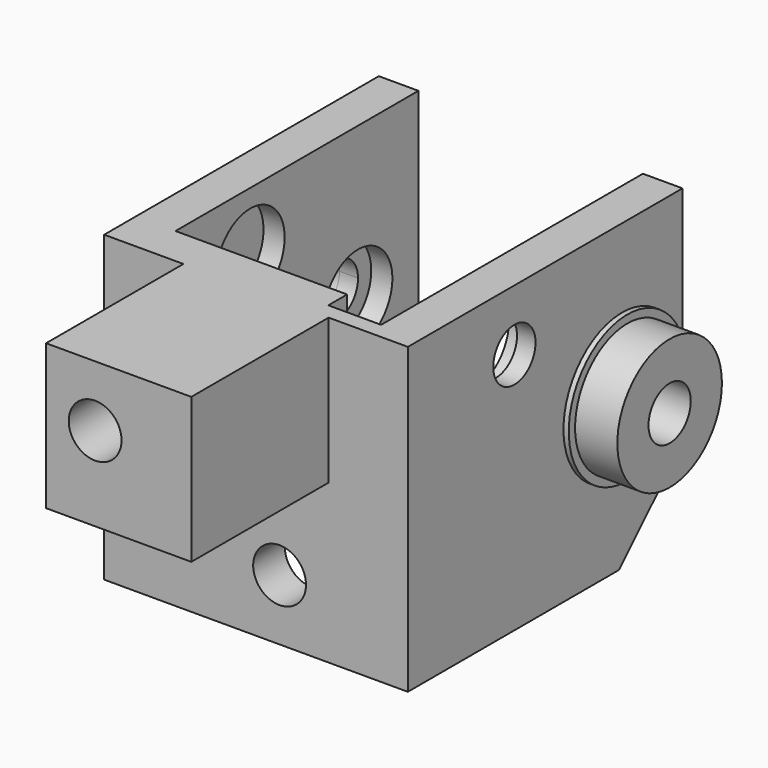
from build123d import *
from build123d import SkipClean  # not in build123d's __all__

# Parameters (mm, degrees)
F1_W             = 115
F1_H             = 115
F2_DEPTH         = 15
F5_W             = 100
F5_H             = 115
F5_R             = 10
F6_DEPTH         = 25
F4_W             = 115
F4_H             = 115
F4_R             = 10
F6_FACE_W        = 25
F6_FACE_H        = 115
F7_DEPTH         = 15
F8_R             = 24.75
F8_R_2           = 10
F9_DEPTH         = 18
F10_SIZE         = 30
F11_R            = 27.75
F11_R_2          = 24.75
F12_DEPTH        = 2
F14_R            = 16.25
F15_DEPTH        = 8
F15_COPIES_COUNT = 2
F15_COPIES_PITCH = 93
F16_R            = 50
F17_DEPTH        = 20
F18_R            = 50
F19_DEPTH        = 20
F20_W            = 115
F20_H            = 115
F20_R            = 10
F21_DEPTH        = 55
F22_W            = 55
F22_H            = 60
F22_R            = 10
F23_DEPTH        = 65


# Not quite as in the source:
# - after a boolean that leaves OpenCascade's solid faulty, fix() repairs it
# - a pattern or mirror of a feature is missing from the dataset's text; its kind, count and spacing are read off the source's solid


with BuildPart() as f2:
    # F1 (on Right) → F2 (new body)
    with BuildSketch(Plane.YZ):
        with Locations((22.08, 34.3903635635)):
            Rectangle(F1_W, F1_H)
        with BuildLine():
            ThreePointArc((8.2903757256, 5.5919290347), (9.5630475596, 2.9237170472), (10, 0))
            ThreePointArc((10, 0), (-9.5630475596, -2.9237170472), (8.2903757256, 5.5919290347))
        make_face(mode=Mode.SUBTRACT)
        with BuildLine():
            ThreePointArc((60.9858107121, 34.3903635635), (53.9095277594, 24.8273160038), (42.6954349866, 28.7984345287))
            ThreePointArc((42.6954349866, 28.7984345287), (48.0620936649, 43.9534111231), (60.9858107121, 34.3903635635))
        make_face(mode=Mode.SUBTRACT)
    extrude(amount=F2_DEPTH)

    # F5 (on face) → F6 (join)
    with BuildSketch(Plane.XZ.offset(35.42)):
        with Locations((50, 34.3903635635)):
            Rectangle(F5_W, F5_H)
        with Locations((66.42, 0)):
            Circle(F5_R, mode=Mode.SUBTRACT)
        with Locations((48.58, 68.7807271269)):
            Circle(F5_R, mode=Mode.SUBTRACT)
    extrude(amount=F6_DEPTH)

    # F4 (on offset) + F6_face (on face) → F7 (join)
    with BuildSketch(Plane.YZ.offset(100)):
        with Locations((22.08, 34.3903635635)):
            Rectangle(F4_W, F4_H)
        with Locations((0, 68.7807271269)):
            Circle(F4_R, mode=Mode.SUBTRACT)
        with Locations((50.9858107121, 34.3903635635)):
            Circle(F4_R, mode=Mode.SUBTRACT)
    with BuildSketch(Plane(origin=(100, -47.92, 34.3903635635), x_dir=(0, 1, 0), z_dir=(1, 0, 0))):
        Rectangle(F6_FACE_W, F6_FACE_H)
    extrude(amount=F7_DEPTH)

    # F8 (on face) → F9 (join)
    with BuildSketch(Plane.YZ):
        with Locations((50.9858107121, 34.3903635635)):
            Circle(F8_R)
        with Locations((50.9858107121, 34.3903635635)):
            Circle(F8_R_2, mode=Mode.SUBTRACT)
    with SkipClean():  # cleaning this boolean's faces spoils the solid; the shape is the same uncleaned
        f9 = extrude(amount=-F9_DEPTH)

    # F9_copies: F9 across plane
    add(f9.mirror(Plane(origin=(57.5, 0, 0), x_dir=(0, 0, 1), z_dir=(1, 0, 0))), clean=False)

    add(f2.part.fix(), mode=Mode.REPLACE)

    # F10
    f10_edges = [f2.edges().sort_by_distance(p)[0] for p in [
        (7.5, 79.58, -23.109636),
        (107.5, 79.58, -23.109636),
    ]]
    chamfer(f10_edges, length=F10_SIZE)

    # F11 (on face) → F12 (join)
    with BuildSketch(Plane.YZ):
        with Locations((50.9858107121, 34.3903635635)):
            Circle(F11_R)
        with Locations((50.9858107121, 34.3903635635)):
            Circle(F11_R_2, mode=Mode.SUBTRACT)
    f12 = extrude(amount=-F12_DEPTH)

    # F12_copies: F12 across plane
    add(f12.mirror(Plane(origin=(57.5, 0, 0), x_dir=(0, 0, 1), z_dir=(1, 0, 0))), clean=False)

    # F14 (on face) → F15 (cut)
    with BuildSketch(Plane(origin=(100, 0, 0), x_dir=(0, -1, 0), z_dir=(-1, 0, 0))):
        with Locations((0, 68.7807271269)):
            Circle(F14_R)
        with Locations((-50.9858107121, 34.3903635635)):
            Circle(F14_R)
        Circle(F14_R)
    f15 = extrude(amount=-F15_DEPTH, mode=Mode.SUBTRACT)

    # F15_copies: F15 ×2
    with SkipClean():  # cleaning this boolean's faces spoils the solid; the shape is the same uncleaned
        with Locations(*[(-i * F15_COPIES_PITCH, 0, 0) for i in range(1, F15_COPIES_COUNT)]):
            add(f15, clean=False, mode=Mode.SUBTRACT)

    # F16 (on face) → F17 (cut)
    with BuildSketch(Plane(origin=(100, 0, 0), x_dir=(0, -1, 0), z_dir=(-1, 0, 0))):
        with Locations((0, 68.7807271269)):
            Circle(F16_R)
    extrude(amount=F17_DEPTH, mode=Mode.SUBTRACT)

    # F18 (on face) → F19 (cut)
    with BuildSketch(Plane.YZ.offset(15)):
        Circle(F18_R)
    extrude(amount=F19_DEPTH, mode=Mode.SUBTRACT)

    # F20 (on face) → F21 (join)
    with BuildSketch(Plane.XZ.offset(60.42)):
        with Locations((57.5, 34.3903635635)):
            Rectangle(F20_W, F20_H)
        with Locations((66.42, 0)):
            Circle(F20_R, mode=Mode.SUBTRACT)
        with Locations((48.58, 68.7807271269)):
            Circle(F20_R, mode=Mode.SUBTRACT)
    extrude(amount=F21_DEPTH)

    # F22 (on face) → F23 (cut)
    with BuildSketch(Plane.XZ.offset(115.42)):
        Polygon((85, 36.8903635635), (85, -23.1096364365), (115, -23.1096364365), (115, 91.8903635635), (85, 91.8903635635), align=None)
        with Locations((57.5, 6.8903635635)):
            Rectangle(F22_W, F22_H)
        with Locations((66.42, 0)):
            Circle(F22_R, mode=Mode.SUBTRACT)
        Polygon((0, -23.1096364365), (30, -23.1096364365), (30, 36.8903635635), (30, 91.8903635635), (0, 91.8903635635), align=None)
    extrude(amount=-F23_DEPTH, mode=Mode.SUBTRACT)


solid = f2.part
